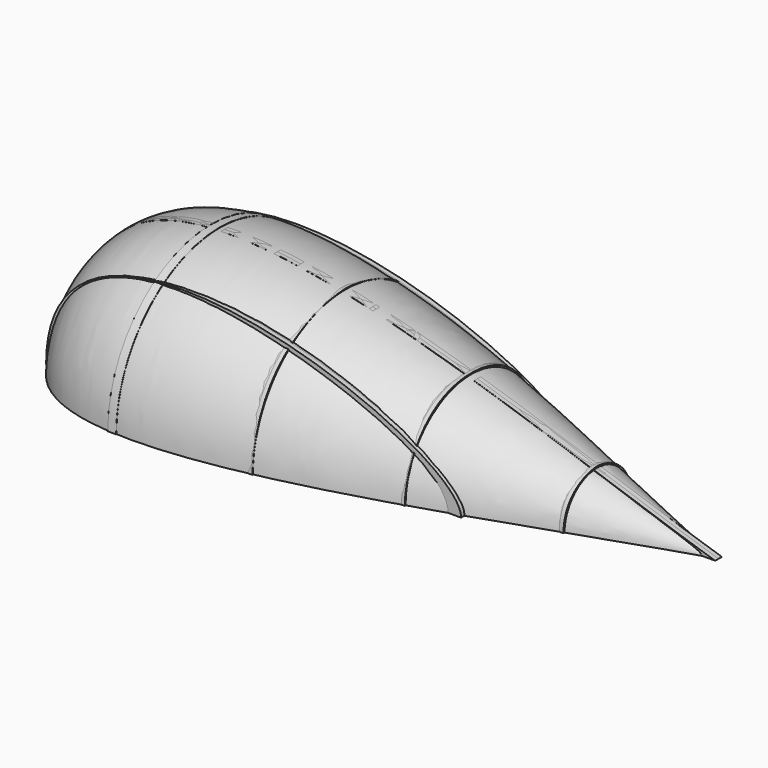
from build123d import *

# Parameters (mm, degrees)
F1_ANGLE_BACK = 90
F1_ANGLE      = 180
F11_DEPTH     = 1
F12_DEPTH     = 1
F13_DEPTH     = 1
F16_DEPTH     = 1


# Not quite as in the source:
# - ends of sketch curves that miss each other by under 0.0002 mm in the source are joined


with BuildPart() as f1:
    # F0 (on Front) → F1 (revolve)
    with BuildSketch(Plane.XZ, mode=Mode.PRIVATE) as f1_sk:
        with BuildLine():
            Line((-75, 0), (0, 0))
            Line((0, 0), (75, 0))
            add(Edge.make_bspline(
                [(-75, 0), (-75, 59.9126815796), (19.3098373711, 17.3266641796), (75, 0)],
                knots=[0, 0, 0, 0, 150, 150, 150, 150], degree=3))
        make_face()
    revolve(f1_sk.sketch.rotate(Axis((-37.5, 0, 0), (-1, 0, 0)), -F1_ANGLE_BACK), axis=Axis((-37.5, 0, 0), (-1, 0, 0)), revolution_arc=F1_ANGLE)


with BuildPart() as f11:
    # F7 (on offset) → F11 (new body, symmetric)
    with BuildSketch(Plane.YZ.offset(-45)):
        with BuildLine():
            add(Edge.make_bspline(
                [(0, 0), (-10.3037776914, 0), (-20.6075553827, 0), (-30.9113330741, 0)],
                knots=[0, 0, 0, 0, 1, 1, 1, 1], degree=3))
            add(Edge.make_bspline(
                [(0, 0), (10.3037776914, 0), (20.6075553827, 0), (30.9113330741, 0)],
                knots=[0, 0, 0, 0, 1, 1, 1, 1], degree=3))
            ThreePointArc((30.9113330741, 0), (0, 30.9113368971), (-30.9113330741, 0))
        make_face()
    extrude(amount=F11_DEPTH, both=True)


with BuildPart() as f12:
    # F8 (on offset) → F12 (new body, symmetric)
    with BuildSketch(Plane.YZ.offset(-15)):
        with BuildLine():
            Line((-27.8169345111, 0), (0, 0))
            Line((0, 0), (27.8169345111, 0))
            add(Edge.make_bspline(
                [(0, 27.8169102967), (5.0467201509, 27.8169102967), (26.5604257584, 24.8144250363), (27.8169345111, 0)],
                knots=[0, 0, 0, 0, 39.339068927, 39.339068927, 39.339068927, 39.339068927], degree=3))
            add(Edge.make_bspline(
                [(0, 27.8169102967), (-5.0467201509, 27.8169102967), (-26.5604257584, 24.8144250363), (-27.8169345111, 0)],
                knots=[0, 0, 0, 0, 39.339068927, 39.339068927, 39.339068927, 39.339068927], degree=3))
        make_face()
    extrude(amount=F12_DEPTH, both=True)


with BuildPart() as f12b:
    # F9 (on offset) → F12, piece 2 (new body, symmetric)
    with BuildSketch(Plane.YZ.offset(15)):
        with BuildLine():
            Line((-19.8365133256, 0), (0, 0))
            Line((0, 0), (19.8365133256, 0))
            add(Edge.make_bspline(
                [(19.8365133256, 0), (19.8365133256, 5.9684109874), (15.1341622695, 19.8365263641), (0, 19.8365263641)],
                knots=[0, 0, 0, 0, 28.0530753948, 28.0530753948, 28.0530753948, 28.0530753948], degree=3))
            add(Edge.make_bspline(
                [(-19.8365133256, 0), (-19.8365133256, 5.9684109874), (-15.1341622695, 19.8365263641), (0, 19.8365263641)],
                knots=[0, 0, 0, 0, 28.0530753948, 28.0530753948, 28.0530753948, 28.0530753948], degree=3))
        make_face()
    extrude(amount=F12_DEPTH, both=True)


with BuildPart() as f12c:
    # F10 (on offset) → F12, piece 3 (new body, symmetric)
    with BuildSketch(Plane.YZ.offset(45)):
        with BuildLine():
            Line((-9.9959000945, 0), (0, 0))
            Line((0, 0), (9.9959000945, 0))
            add(Edge.make_bspline(
                [(0, 9.9958991632), (3.0557271093, 9.9958991632), (9.9959000945, 7.6686600223), (9.9959000945, 0)],
                knots=[0, 0, 0, 0, 14.1363368232, 14.1363368232, 14.1363368232, 14.1363368232], degree=3))
            add(Edge.make_bspline(
                [(0, 9.9958991632), (-3.0557271093, 9.9958991632), (-9.9959000945, 7.6686600223), (-9.9959000945, 0)],
                knots=[0, 0, 0, 0, 14.1363368232, 14.1363368232, 14.1363368232, 14.1363368232], degree=3))
        make_face()
    extrude(amount=F12_DEPTH, both=True)


with BuildPart() as f13:
    # F0 (on Front) → F13 (new body, symmetric)
    with BuildSketch(Plane.XZ):
        with BuildLine():
            Line((-75, 0), (0, 0))
            Line((0, 0), (75, 0))
            add(Edge.make_bspline(
                [(-75, 0), (-75, 59.9126815796), (19.3098373711, 17.3266641796), (75, 0)],
                knots=[0, 0, 0, 0, 150, 150, 150, 150], degree=3))
        make_face()
    extrude(amount=F13_DEPTH, both=True)


with BuildPart() as f16:
    # F15 (on offset) → F16 (new body, symmetric)
    with BuildSketch(Plane.XZ.offset(-16)):
        with BuildLine():
            Line((-71.8375742435, 0), (27.1770562977, 0))
            add(Edge.make_bspline(
                [(27.1770562977, 0), (27.1770562977, 15.0069938973), (-71.8375742435, 50.7412180305), (-71.8375742435, 0)],
                knots=[0, 0, 0, 0, 99.0146305412, 99.0146305412, 99.0146305412, 99.0146305412], degree=3))
        make_face()
    extrude(amount=F16_DEPTH, both=True)


with BuildPart() as f17_1:
    # F17: instance of F16
    add(f16.part.mirror(Plane.XZ))


solid = Compound([f1.part, f11.part, f12.part, f12b.part, f12c.part, f13.part, f16.part, f17_1.part])
